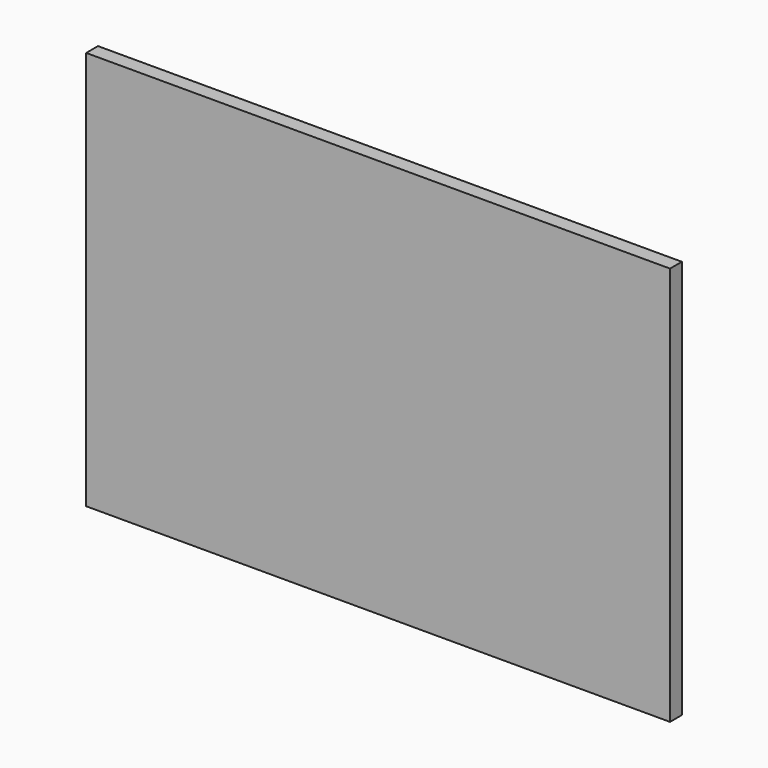
from build123d import *

# Parameters (mm, degrees)
F0_W     = 250.825
F0_H     = 171.45
F1_DEPTH = 6.35


# Not quite as in the source:
# - a length typed as a fraction of an inch, garbled in the dataset ("3 / 203.2 mm" for 3/8 in), is restored


with BuildPart() as f1:
    # F0 (on Front) → F1 (new body)
    with BuildSketch(Plane.XZ):
        Rectangle(F0_W, F0_H)
    extrude(amount=F1_DEPTH)


solid = f1.part
